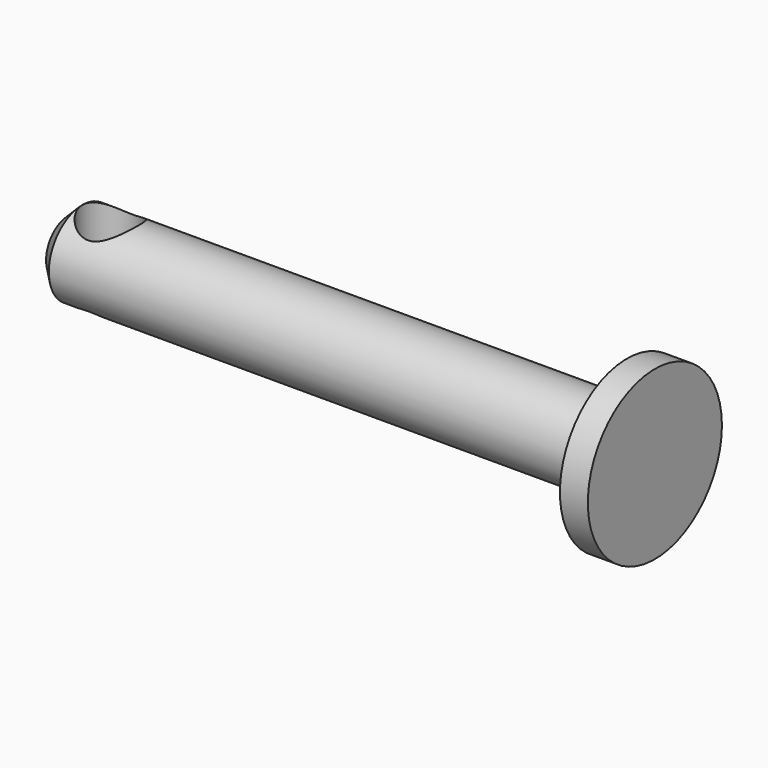
from build123d import *

# Parameters (mm, degrees)
F2_R     = 4
F3_DEPTH = 12.5
F4_SIZE  = 1.99999


# Not quite as in the source:
# - a fillet or chamfer is up to 0.001 mm smaller than in the source, because OpenCascade refuses the exact size


with BuildPart() as f1:
    # F0 (on Top) → F1 (revolve)
    with BuildSketch(Plane.XY):
        Polygon((0, 6), (0, 0), (84, 0), (84, 12), (80, 12), (80, 6), align=None)
    revolve(axis=Axis((42, 0, 0), (1, 0, 0)))

    # F2 (on Top) → F3 (cut, symmetric)
    with BuildSketch(Plane.XY):
        with Locations((6, 0)):
            Circle(F2_R)
    extrude(amount=F3_DEPTH, both=True, mode=Mode.SUBTRACT)

    # F4 (size 2 in the source; OpenCascade refuses exactly that, so slightly less here)
    f4_edges = [f1.edges().sort_by_distance(p)[0] for p in [
        (0, -6, 0),
    ]]
    chamfer(f4_edges, length=F4_SIZE)


solid = f1.part
